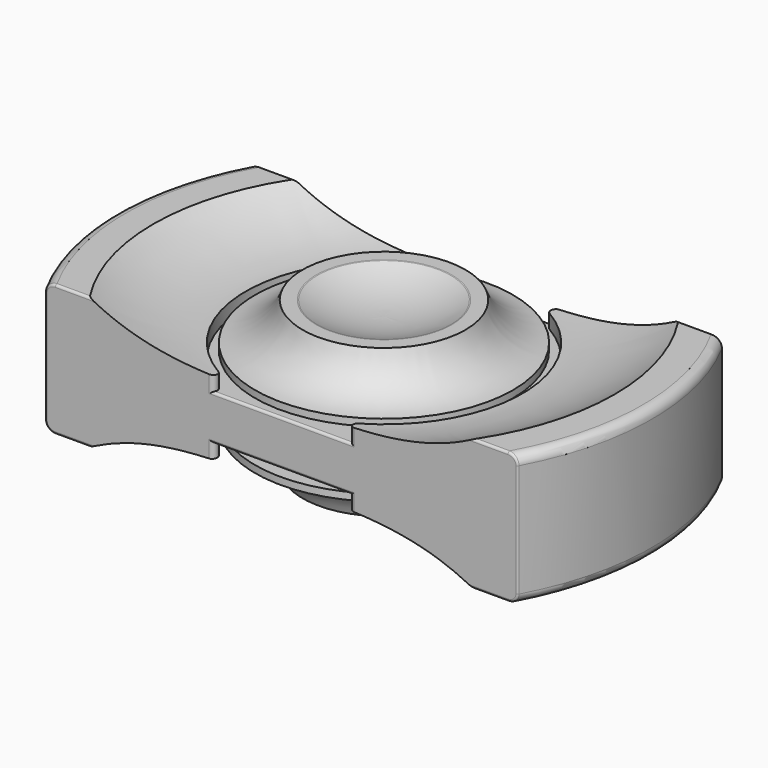
from build123d import *

# Parameters (mm, degrees)
F3_DEPTH = 12.5
F4_R     = 1
F5_R     = 0.5
F6_R     = 0.25
F6_2_R   = 0.25
F8_DEPTH = 25
F9_R     = 5
F10_R    = 1
F11_R    = 0.25


with BuildPart() as f1:
    # F0 (on Front) → F1 (revolve)
    with BuildSketch(Plane.XZ):
        with BuildLine():
            Line((6.35, 4.7625), (6.35, 0))
            Line((6.35, 0), (12.7, 0))
            Line((12.7, 0), (14.7, 0))
            Line((14.7, 0), (14.7, -1.5))
            ThreePointArc((14.7, -1.5), (19.8103903429, -2.398268672), (24.5, -4.61875))
            Line((24.5, -4.61875), (28.5, -4.61875))
            Line((28.5, -4.61875), (28.5, 2.38125))
            Line((28.5, 2.38125), (28.5, 9.38125))
            Line((28.5, 9.38125), (24.5, 9.38125))
            ThreePointArc((24.5, 9.38125), (19.8103903429, 7.160768672), (14.7, 6.2625))
            Line((14.7, 6.2625), (14.7, 4.7625))
            Line((14.7, 4.7625), (12.7, 4.7625))
            Line((12.7, 4.7625), (6.35, 4.7625))
        make_face()
    revolve(axis=Axis((0, 0, 2.38125), (0, 0, 1)))

    # F2 (on Top) → F3 (cut, symmetric)
    with BuildSketch(Plane.XY):
        Polygon((34.263856709, -13.6), (13.6, -13.6), (-13.6, -13.6), (-29.1756652296, -13.6), (-29.1756652296, -33.6904525757), (34.263856709, -33.6904525757), align=None)
        Polygon((-13.6, 13.6), (13.6, 13.6), (32.8008905053, 13.6), (32.8008905053, 33.2069918513), (-29.3086618185, 33.2069918513), (-29.3086618185, 13.6), align=None)
    extrude(amount=F3_DEPTH, both=True, mode=Mode.SUBTRACT)

    # F4
    f4_edges = [f1.edges().sort_by_distance(p)[0] for p in [
        (28.5, 0, -4.61875),
        (-28.5, 0, -4.61875),
        (28.5, 0, 9.38125),
        (-28.5, 0, 9.38125),
    ]]
    fillet(f4_edges, radius=F4_R)

    # F5
    f5_edges = [f1.edges().sort_by_distance(p)[0] for p in [
        (-5.579426, 13.6, -0.75),
        (5.579426, 13.6, -0.75),
        (5.579426, 13.6, 5.5125),
        (-5.579426, 13.6, 5.5125),
        (-5.579426, -13.6, -0.75),
        (5.579426, -13.6, -0.75),
        (5.579426, -13.6, 5.5125),
        (-5.579426, -13.6, 5.5125),
    ]]
    fillet(f5_edges, radius=F5_R)

    # F6
    f6_edges = [f1.edges().sort_by_distance(p)[0] for p in [
        (25.045758, -13.6, 2.38125),
        (-25.045758, -13.6, 2.38125),
        (25.045758, 13.6, 2.38125),
        (-25.045758, 13.6, 2.38125),
        (0, -13.6, 0),
        (0, -13.6, 4.7625),
        (0, 13.6, 0),
        (0, 13.6, 4.7625),
    ]]
    fillet(f6_edges, radius=F6_R)

    # F7 (on face) → F8 (cut)
    with BuildSketch(Plane.XY.offset(4.7625)):
        with BuildLine():
            ThreePointArc((-6.4411438468, 10.9453947368), (-12.7, 0), (-6.4411438468, -10.9453947368))
            Line((-6.4411438468, -10.9453947368), (-2, -10.9453947368))
            Line((-2, -10.9453947368), (-2, -8.1069414701))
            ThreePointArc((-2, -8.1069414701), (-8.35, 0), (-2, 8.1069414701))
            Line((-2, 8.1069414701), (-2, 10.9453947368))
            Line((-2, 10.9453947368), (-6.4411438468, 10.9453947368))
        make_face()
        with BuildLine():
            Line((2, -10.9453947368), (6.4411438468, -10.9453947368))
            ThreePointArc((6.4411438468, -10.9453947368), (12.7, 0), (6.4411438468, 10.9453947368))
            Line((6.4411438468, 10.9453947368), (2, 10.9453947368))
            Line((2, 10.9453947368), (2, 8.1069414701))
            ThreePointArc((2, 8.1069414701), (8.35, 0), (2, -8.1069414701))
            Line((2, -8.1069414701), (2, -10.9453947368))
        make_face()
    extrude(amount=-F8_DEPTH, mode=Mode.SUBTRACT)

    # F9
    f9_edges = [f1.edges().sort_by_distance(p)[0] for p in [
        (6.441144, 10.945395, 2.38125),
        (-6.441144, 10.945395, 2.38125),
        (-6.441144, -10.945395, 2.38125),
        (6.441144, -10.945395, 2.38125),
    ]]
    fillet(f9_edges, radius=F9_R)

    # F10
    f10_edges = [f1.edges().sort_by_distance(p)[0] for p in [
        (-2, 10.945395, 2.38125),
        (2, 8.106941, 2.38125),
        (2, -10.945395, 2.38125),
        (-2, 8.106941, 2.38125),
        (2, 10.945395, 2.38125),
        (2, -8.106941, 2.38125),
        (-2, -10.945395, 2.38125),
        (-2, -8.106941, 2.38125),
    ]]
    fillet(f10_edges, radius=F10_R)


with BuildPart() as f1b:
    # F0 (on Front) → F1, piece 2 (revolve)
    with BuildSketch(Plane.XZ):
        with BuildLine():
            Line((0, 8.6944758326), (0, 6.2577016652))
            Line((0, 6.2577016652), (0, 5.5101008326))
            Line((0, 5.5101008326), (0, 4.7625))
            Line((0, 4.7625), (0, 0))
            Line((0, 0), (3.175, 0))
            Line((3.175, 0), (3.175, 4.7625))
            Line((3.175, 4.7625), (4.3, 4.7625))
            Line((4.3, 4.7625), (4.3, 5.5101008326))
            Line((4.3, 5.5101008326), (12.7, 5.5101008326))
            Line((12.7, 5.5101008326), (13.7, 5.5101008326))
            Line((13.7, 5.5101008326), (13.7, 6.2625))
            ThreePointArc((13.7, 6.2625), (10.5806584202, 7.5069279194), (8.6518969432, 10.25625))
            Line((8.6518969432, 10.25625), (7.1356836706, 10.25625))
            ThreePointArc((7.1356836706, 10.25625), (3.6623889041, 9.0433811427), (0, 8.6944758326))
        make_face()
    revolve(axis=Axis((0, 0, 2.38125), (0, 0, 1)))

    # F11
    f11_edges = [f1b.edges().sort_by_distance(p)[0] for p in [
        (-7.135684, 0, 10.25625),
    ]]
    fillet(f11_edges, radius=F11_R)


with BuildPart() as f1c:
    # F0 (on Front) → F1, piece 3 (revolve)
    with BuildSketch(Plane.XZ):
        with BuildLine():
            Line((13.7, -0.7476008326), (12.7, -0.7476008326))
            Line((12.7, -0.7476008326), (0, -0.7476008326))
            Line((0, -0.7476008326), (0, -3.9319758326))
            ThreePointArc((0, -3.9319758326), (3.6623889041, -4.2808811427), (7.1356836706, -5.49375))
            Line((7.1356836706, -5.49375), (8.6518969432, -5.49375))
            ThreePointArc((8.6518969432, -5.49375), (10.5806584202, -2.7444279194), (13.7, -1.5))
            Line((13.7, -1.5), (13.7, -0.7476008326))
        make_face()
    revolve(axis=Axis((0, 0, 2.38125), (0, 0, 1)))

    # F6#2
    f6_2_edges = [f1c.edges().sort_by_distance(p)[0] for p in [
        (-7.135684, 0, -5.49375),
    ]]
    fillet(f6_2_edges, radius=F6_2_R)


solid = Compound([f1.part, f1b.part, f1c.part])
